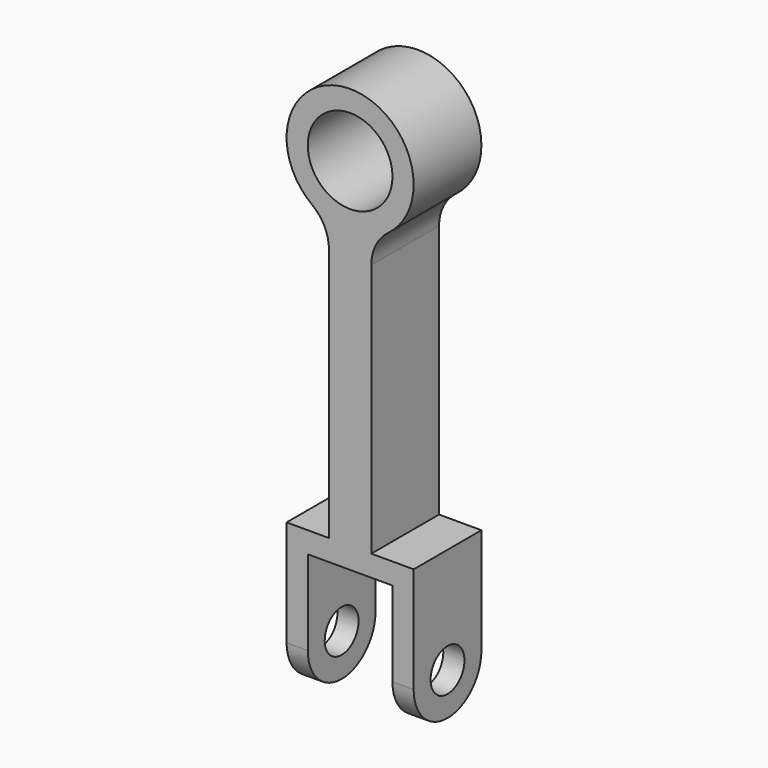
from build123d import *

# Parameters (mm, degrees)
F0_R     = 25.4
F1_DEPTH = 25.4
F2_R     = 25.39999
F3_R     = 12.7
F4_DEPTH = 12.7
F5_R     = 12.7
F6_DEPTH = 12.7


# Not quite as in the source:
# - a fillet or chamfer is up to 0.001 mm smaller than in the source, because OpenCascade refuses the exact size


with BuildPart() as f1:
    # F0 (on Front) → F1 (new body, symmetric)
    with BuildSketch(Plane.XZ):
        with BuildLine():
            ThreePointArc((12.7, -35.9210244843), (31.1085197333, -21.9970452561), (38.1, 0))
            ThreePointArc((38.1, 0), (-21.9970452561, 31.1085197333), (-12.7, -35.9210244843))
            ThreePointArc((-12.7, -35.9210244843), (0, -38.1), (12.7, -35.9210244843))
        make_face()
        Circle(F0_R, mode=Mode.SUBTRACT)
        with BuildLine():
            ThreePointArc((12.7, -35.9210244843), (0, -38.1), (-12.7, -35.9210244843))
            Line((-12.7, -35.9210244843), (-12.7, -203.2))
            Line((-12.7, -203.2), (-38.1, -203.2))
            Line((-38.1, -203.2), (-38.1, -292.1))
            Line((-38.1, -292.1), (-25.4, -292.1))
            Line((-25.4, -292.1), (-25.4, -215.9))
            Line((-25.4, -215.9), (25.4, -215.9))
            Line((25.4, -215.9), (25.4, -292.1))
            Line((25.4, -292.1), (38.1, -292.1))
            Line((38.1, -292.1), (38.1, -203.2))
            Line((38.1, -203.2), (12.7, -203.2))
            Line((12.7, -203.2), (12.7, -35.9210244843))
        make_face()
    extrude(amount=F1_DEPTH, both=True)

    # F2 (radius 25.4 in the source; OpenCascade refuses exactly that, so slightly less here)
    f2_edges = [f1.edges().sort_by_distance(p)[0] for p in [
        (12.7, 0, -35.921024),
        (-12.7, 0, -35.921024),
        (-31.75, -25.4, -292.1),
        (-31.75, 25.4, -292.1),
        (31.75, -25.4, -292.1),
        (31.75, 25.4, -292.1),
    ]]
    fillet(f2_edges, radius=F2_R)

    # F3 (on face) → F4 (cut, through all)
    with BuildSketch(Plane(origin=(-38.1, 0, 0), x_dir=(0, -1, 0), z_dir=(-1, 0, 0))):
        with Locations((0, -266.7)):
            Circle(F3_R)
    extrude(amount=-F4_DEPTH, mode=Mode.SUBTRACT)

    # F5 (on face) → F6 (cut, through all)
    with BuildSketch(Plane.YZ.offset(38.1)):
        with Locations((0, -266.7)):
            Circle(F5_R)
    extrude(amount=-F6_DEPTH, mode=Mode.SUBTRACT)


solid = f1.part
